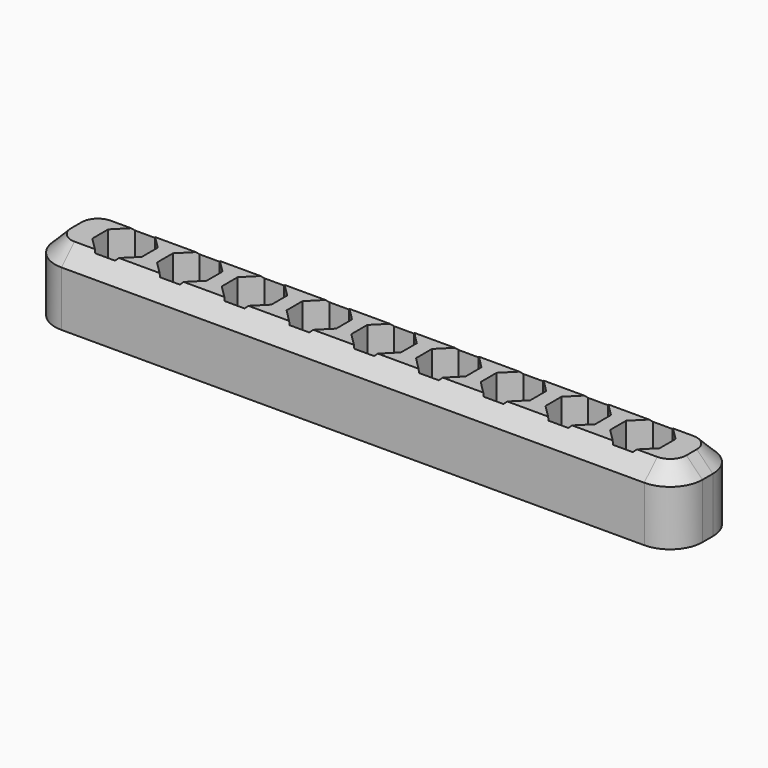
from build123d import *

# Parameters (mm, degrees)
F0_W         = 100
F0_H         = 12
F1_DEPTH     = 11
F0_W_2       = 2.3021356216
F0_H_2       = 3.0731172886
F0_W_3       = 3.0519974387
F0_H_3       = 2.2957974076
F2_DEPTH     = 1
F3_R         = 5
F4_T1_DEPTH  = 90
F4_T3_DEPTH  = 2
F4_T6_ANGLE  = 90
F4_T8_ANGLE  = 90
F4_T10_ANGLE = 90
F4_T12_ANGLE = 90


# Not quite as in the source:
# - a fillet or chamfer that OpenCascade refuses, or shapes differently, is made with other operations: its cross-section is extruded or revolved along the edge and cut away or added


with BuildPart() as f1:
    # F0 (on Top) → F1 (new body)
    with BuildSketch(Plane.XY):
        Rectangle(F0_W, F0_H)
        Polygon((-43.828134341, 1.5365586443), (-41.5259987194, 3.8323560519), (-38.4740012806, 3.8323560519), (-36.171865659, 1.5365586443), (-36.171865659, -1.5365586443), (-38.4740012806, -3.8323560519), (-41.5259987194, -3.8323560519), (-43.828134341, -1.5365586443), align=None, mode=Mode.SUBTRACT)
        Polygon((-13.8175263533, 1.5313583214), (-11.5153907317, 3.827155729), (-8.463393293, 3.827155729), (-6.1612576714, 1.5313583214), (-6.1612576714, -1.5417589672), (-8.463393293, -3.8375563748), (-11.5153907317, -3.8375563748), (-13.8175263533, -1.5417589672), align=None, mode=Mode.SUBTRACT)
        Polygon((6.1764764136, 1.531357914), (8.4786120352, 3.8271553215), (11.5306094739, 3.8271553215), (13.8327450955, 1.531357914), (13.8327450955, -1.5417593747), (11.5306094739, -3.8375567823), (8.4786120352, -3.8375567823), (6.1764764136, -1.5417593747), align=None, mode=Mode.SUBTRACT)
        Polygon((36.1682959368, 1.5178143587), (38.4704315585, 3.8136117663), (41.5224289972, 3.8136117663), (43.8245646188, 1.5178143587), (43.8245646188, -1.5553029299), (41.5224289972, -3.8511003375), (38.4704315585, -3.8511003375), (36.1682959368, -1.5553029299), align=None, mode=Mode.SUBTRACT)
        Polygon((-33.8281344609, 1.5365587602), (-31.5259988393, 3.8323561678), (-28.4740014006, 3.8323561678), (-26.1718657789, 1.5365587602), (-26.1718657789, -1.5365585284), (-28.4740014006, -3.832355936), (-31.5259988393, -3.832355936), (-33.8281344609, -1.5365585284), align=None, mode=Mode.SUBTRACT)
        Polygon((-23.8324813077, 1.5400278102), (-21.5303456861, 3.8358252178), (-18.4783482474, 3.8358252178), (-16.1762126258, 1.5400278102), (-16.1762126258, -1.5330894784), (-18.4783482474, -3.828886886), (-21.5303456861, -3.828886886), (-23.8324813077, -1.5330894784), align=None, mode=Mode.SUBTRACT)
        Polygon((-3.8348879394, 1.5600861226), (-1.5327523178, 3.8558835302), (1.5192451209, 3.8558835302), (3.8213807426, 1.5600861226), (3.8213807426, -1.513031166), (1.5192451209, -3.8088285736), (-1.5327523178, -3.8088285736), (-3.8348879394, -1.513031166), align=None, mode=Mode.SUBTRACT)
        Polygon((16.1591154059, 1.5457221845), (18.4612510276, 3.8415195921), (21.5132484663, 3.8415195921), (23.8153840879, 1.5457221845), (23.8153840879, -1.5273951041), (21.5132484663, -3.8231925117), (18.4612510276, -3.8231925117), (16.1591154059, -1.5273951041), align=None, mode=Mode.SUBTRACT)
        Polygon((26.1708870998, 1.5457229285), (28.4730227214, 3.8415203361), (31.5250201601, 3.8415203361), (33.8271557817, 1.5457229285), (33.8271557817, -1.5273943601), (31.5250201601, -3.8231917677), (28.4730227214, -3.8231917677), (26.1708870998, -1.5273943601), align=None, mode=Mode.SUBTRACT)
    extrude(amount=F1_DEPTH)

    # F0 (on Top) → F2 (join)
    with BuildSketch(Plane.XY):
        Rectangle(F0_W, F0_H)
        Polygon((-43.828134341, 1.5365586443), (-41.5259987194, 3.8323560519), (-38.4740012806, 3.8323560519), (-36.171865659, 1.5365586443), (-36.171865659, -1.5365586443), (-38.4740012806, -3.8323560519), (-41.5259987194, -3.8323560519), (-43.828134341, -1.5365586443), align=None, mode=Mode.SUBTRACT)
        Polygon((-13.8175263533, 1.5313583214), (-11.5153907317, 3.827155729), (-8.463393293, 3.827155729), (-6.1612576714, 1.5313583214), (-6.1612576714, -1.5417589672), (-8.463393293, -3.8375563748), (-11.5153907317, -3.8375563748), (-13.8175263533, -1.5417589672), align=None, mode=Mode.SUBTRACT)
        Polygon((6.1764764136, 1.531357914), (8.4786120352, 3.8271553215), (11.5306094739, 3.8271553215), (13.8327450955, 1.531357914), (13.8327450955, -1.5417593747), (11.5306094739, -3.8375567823), (8.4786120352, -3.8375567823), (6.1764764136, -1.5417593747), align=None, mode=Mode.SUBTRACT)
        Polygon((36.1682959368, 1.5178143587), (38.4704315585, 3.8136117663), (41.5224289972, 3.8136117663), (43.8245646188, 1.5178143587), (43.8245646188, -1.5553029299), (41.5224289972, -3.8511003375), (38.4704315585, -3.8511003375), (36.1682959368, -1.5553029299), align=None, mode=Mode.SUBTRACT)
        Polygon((-33.8281344609, 1.5365587602), (-31.5259988393, 3.8323561678), (-28.4740014006, 3.8323561678), (-26.1718657789, 1.5365587602), (-26.1718657789, -1.5365585284), (-28.4740014006, -3.832355936), (-31.5259988393, -3.832355936), (-33.8281344609, -1.5365585284), align=None, mode=Mode.SUBTRACT)
        Polygon((-23.8324813077, 1.5400278102), (-21.5303456861, 3.8358252178), (-18.4783482474, 3.8358252178), (-16.1762126258, 1.5400278102), (-16.1762126258, -1.5330894784), (-18.4783482474, -3.828886886), (-21.5303456861, -3.828886886), (-23.8324813077, -1.5330894784), align=None, mode=Mode.SUBTRACT)
        Polygon((-3.8348879394, 1.5600861226), (-1.5327523178, 3.8558835302), (1.5192451209, 3.8558835302), (3.8213807426, 1.5600861226), (3.8213807426, -1.513031166), (1.5192451209, -3.8088285736), (-1.5327523178, -3.8088285736), (-3.8348879394, -1.513031166), align=None, mode=Mode.SUBTRACT)
        Polygon((16.1591154059, 1.5457221845), (18.4612510276, 3.8415195921), (21.5132484663, 3.8415195921), (23.8153840879, 1.5457221845), (23.8153840879, -1.5273951041), (21.5132484663, -3.8231925117), (18.4612510276, -3.8231925117), (16.1591154059, -1.5273951041), align=None, mode=Mode.SUBTRACT)
        Polygon((26.1708870998, 1.5457229285), (28.4730227214, 3.8415203361), (31.5250201601, 3.8415203361), (33.8271557817, 1.5457229285), (33.8271557817, -1.5273943601), (31.5250201601, -3.8231917677), (28.4730227214, -3.8231917677), (26.1708870998, -1.5273943601), align=None, mode=Mode.SUBTRACT)
        with Locations((-42.6770665302, 0)):
            Rectangle(F0_W_2, F0_H_2)
        Polygon((-41.5259987194, 1.5365586443), (-41.5259987194, 3.8323560519), (-43.828134341, 1.5365586443), align=None)
        with Locations((-40, 2.6844573481)):
            Rectangle(F0_W_3, F0_H_3)
        Polygon((-41.5259987194, -3.8323560519), (-41.5259987194, -1.5365586443), (-43.828134341, -1.5365586443), align=None)
        with Locations((-40, -2.6844573481)):
            Rectangle(F0_W_3, F0_H_3)
        with Locations((-40, 0)):
            Rectangle(F0_W_3, F0_H_2)
        with Locations((-37.3229334698, 0)):
            Rectangle(F0_W_2, F0_H_2)
        Polygon((-36.171865659, 1.5365586443), (-38.4740012806, 3.8323560519), (-38.4740012806, 1.5365586443), align=None)
        Polygon((-36.171865659, -1.5365586443), (-38.4740012806, -1.5365586443), (-38.4740012806, -3.8323560519), align=None)
        Polygon((-31.5259988393, -3.832355936), (-31.5259988393, -1.5365585284), (-33.8281344609, -1.5365585284), align=None)
        with Locations((-32.6770666501, 1.159e-07)):
            Rectangle(F0_W_2, F0_H_2)
        Polygon((-31.5259988393, 1.5365587602), (-31.5259988393, 3.8323561678), (-33.8281344609, 1.5365587602), align=None)
        with Locations((-30.0000001199, 2.684457464)):
            Rectangle(F0_W_3, F0_H_3)
        Polygon((-26.1718657789, 1.5365587602), (-28.4740014006, 3.8323561678), (-28.4740014006, 1.5365587602), align=None)
        with Locations((-27.3229335898, 1.159e-07)):
            Rectangle(F0_W_2, F0_H_2)
        with Locations((-30.0000001199, 1.159e-07)):
            Rectangle(F0_W_3, F0_H_2)
        with Locations((-30.0000001199, -2.6844572322)):
            Rectangle(F0_W_3, F0_H_3)
        Polygon((-26.1718657789, -1.5365585284), (-28.4740014006, -1.5365585284), (-28.4740014006, -3.832355936), align=None)
        Polygon((-21.5303456861, -3.828886886), (-21.5303456861, -1.5330894784), (-23.8324813077, -1.5330894784), align=None)
        with Locations((-22.6814134969, 0.0034691659)):
            Rectangle(F0_W_2, F0_H_2)
        Polygon((-21.5303456861, 1.5400278102), (-21.5303456861, 3.8358252178), (-23.8324813077, 1.5400278102), align=None)
        with Locations((-20.0043469667, 2.687926514)):
            Rectangle(F0_W_3, F0_H_3)
        with Locations((-20.0043469667, 0.0034691659)):
            Rectangle(F0_W_3, F0_H_2)
        with Locations((-20.0043469667, -2.6809881822)):
            Rectangle(F0_W_3, F0_H_3)
        Polygon((-16.1762126258, -1.5330894784), (-18.4783482474, -1.5330894784), (-18.4783482474, -3.828886886), align=None)
        with Locations((-17.3272804366, 0.0034691659)):
            Rectangle(F0_W_2, F0_H_2)
        Polygon((-16.1762126258, 1.5400278102), (-18.4783482474, 3.8358252178), (-18.4783482474, 1.5400278102), align=None)
        Polygon((-11.5153907317, 1.5313583214), (-11.5153907317, 3.827155729), (-13.8175263533, 1.5313583214), align=None)
        with Locations((-12.6664585425, -0.0052003229)):
            Rectangle(F0_W_2, F0_H_2)
        Polygon((-11.5153907317, -3.8375563748), (-11.5153907317, -1.5417589672), (-13.8175263533, -1.5417589672), align=None)
        with Locations((-9.9893920124, -2.689657671)):
            Rectangle(F0_W_3, F0_H_3)
        with Locations((-9.9893920124, 2.6792570252)):
            Rectangle(F0_W_3, F0_H_3)
        with Locations((-7.3123254822, -0.0052003229)):
            Rectangle(F0_W_2, F0_H_2)
        Polygon((-6.1612576714, 1.5313583214), (-8.463393293, 3.827155729), (-8.463393293, 1.5313583214), align=None)
        Polygon((-6.1612576714, -1.5417589672), (-8.463393293, -1.5417589672), (-8.463393293, -3.8375563748), align=None)
        with Locations((-9.9893920124, -0.0052003229)):
            Rectangle(F0_W_3, F0_H_2)
        Polygon((-1.5327523178, 1.5600861226), (-1.5327523178, 3.8558835302), (-3.8348879394, 1.5600861226), align=None)
        with Locations((-0.0067535984, 2.7079848264)):
            Rectangle(F0_W_3, F0_H_3)
        Polygon((3.8213807426, 1.5600861226), (1.5192451209, 3.8558835302), (1.5192451209, 1.5600861226), align=None)
        with Locations((2.6703129317, 0.0235274783)):
            Rectangle(F0_W_2, F0_H_2)
        with Locations((-0.0067535984, 0.0235274783)):
            Rectangle(F0_W_3, F0_H_2)
        with Locations((-2.6838201286, 0.0235274783)):
            Rectangle(F0_W_2, F0_H_2)
        with Locations((-0.0067535984, -2.6609298698)):
            Rectangle(F0_W_3, F0_H_3)
        Polygon((3.8213807426, -1.513031166), (1.5192451209, -1.513031166), (1.5192451209, -3.8088285736), align=None)
        Polygon((-1.5327523178, -3.8088285736), (-1.5327523178, -1.513031166), (-3.8348879394, -1.513031166), align=None)
        with Locations((7.3275442244, -0.0052007304)):
            Rectangle(F0_W_2, F0_H_2)
        Polygon((8.4786120352, 1.531357914), (8.4786120352, 3.8271553215), (6.1764764136, 1.531357914), align=None)
        with Locations((10.0046107545, 2.6792566177)):
            Rectangle(F0_W_3, F0_H_3)
        Polygon((13.8327450955, 1.531357914), (11.5306094739, 3.8271553215), (11.5306094739, 1.531357914), align=None)
        with Locations((12.6816772847, -0.0052007304)):
            Rectangle(F0_W_2, F0_H_2)
        with Locations((10.0046107545, -0.0052007304)):
            Rectangle(F0_W_3, F0_H_2)
        Polygon((8.4786120352, -3.8375567823), (8.4786120352, -1.5417593747), (6.1764764136, -1.5417593747), align=None)
        with Locations((10.0046107545, -2.6896580785)):
            Rectangle(F0_W_3, F0_H_3)
        Polygon((13.8327450955, -1.5417593747), (11.5306094739, -1.5417593747), (11.5306094739, -3.8375567823), align=None)
        with Locations((17.3101832167, 0.0091635402)):
            Rectangle(F0_W_2, F0_H_2)
        Polygon((18.4612510276, -3.8231925117), (18.4612510276, -1.5273951041), (16.1591154059, -1.5273951041), align=None)
        with Locations((19.9872497469, -2.6752938079)):
            Rectangle(F0_W_3, F0_H_3)
        Polygon((23.8153840879, -1.5273951041), (21.5132484663, -1.5273951041), (21.5132484663, -3.8231925117), align=None)
        with Locations((22.6643162771, 0.0091635402)):
            Rectangle(F0_W_2, F0_H_2)
        with Locations((19.9872497469, 0.0091635402)):
            Rectangle(F0_W_3, F0_H_2)
        with Locations((19.9872497469, 2.6936208883)):
            Rectangle(F0_W_3, F0_H_3)
        Polygon((18.4612510276, 1.5457221845), (18.4612510276, 3.8415195921), (16.1591154059, 1.5457221845), align=None)
        Polygon((23.8153840879, 1.5457221845), (21.5132484663, 3.8415195921), (21.5132484663, 1.5457221845), align=None)
        Polygon((28.4730227214, 1.5457229285), (28.4730227214, 3.8415203361), (26.1708870998, 1.5457229285), align=None)
        with Locations((27.3219549106, 0.0091642842)):
            Rectangle(F0_W_2, F0_H_2)
        Polygon((28.4730227214, -3.8231917677), (28.4730227214, -1.5273943601), (26.1708870998, -1.5273943601), align=None)
        with Locations((29.9990214407, -2.6752930639)):
            Rectangle(F0_W_3, F0_H_3)
        with Locations((29.9990214407, 0.0091642842)):
            Rectangle(F0_W_3, F0_H_2)
        with Locations((29.9990214407, 2.6936216323)):
            Rectangle(F0_W_3, F0_H_3)
        Polygon((33.8271557817, 1.5457229285), (31.5250201601, 3.8415203361), (31.5250201601, 1.5457229285), align=None)
        with Locations((32.6760879709, 0.0091642842)):
            Rectangle(F0_W_2, F0_H_2)
        Polygon((33.8271557817, -1.5273943601), (31.5250201601, -1.5273943601), (31.5250201601, -3.8231917677), align=None)
        with Locations((37.3193637477, -0.0187442856)):
            Rectangle(F0_W_2, F0_H_2)
        Polygon((38.4704315585, -3.8511003375), (38.4704315585, -1.5553029299), (36.1682959368, -1.5553029299), align=None)
        with Locations((39.9964302778, -2.7032016337)):
            Rectangle(F0_W_3, F0_H_3)
        with Locations((42.673496808, -0.0187442856)):
            Rectangle(F0_W_2, F0_H_2)
        with Locations((39.9964302778, 2.6657130625)):
            Rectangle(F0_W_3, F0_H_3)
        Polygon((38.4704315585, 1.5178143587), (38.4704315585, 3.8136117663), (36.1682959368, 1.5178143587), align=None)
        with Locations((39.9964302778, -0.0187442856)):
            Rectangle(F0_W_3, F0_H_2)
        Polygon((43.8245646188, 1.5178143587), (41.5224289972, 3.8136117663), (41.5224289972, 1.5178143587), align=None)
        Polygon((43.8245646188, -1.5553029299), (41.5224289972, -1.5553029299), (41.5224289972, -3.8511003375), align=None)
    extrude(amount=F2_DEPTH)

    # F3
    f3_edges = [f1.edges().sort_by_distance(p)[0] for p in [
        (-50, 6, 5.5),
        (50, -6, 5.5),
        (50, 6, 5.5),
        (-50, -6, 5.5),
    ]]
    fillet(f3_edges, radius=F3_R)

    # F4: chamfer of 2.5 on 8 edges, made by hand

    # F4_s2 → F4_t1 (cut)
    with BuildSketch(Plane.YZ.offset(-45)):
        Polygon((-6, 8.5), (-3.5, 11), (-6, 11), align=None)
        Polygon((3.5, 11), (6, 8.5), (6, 11), align=None)
    extrude(amount=F4_T1_DEPTH, mode=Mode.SUBTRACT)

    # F4_s4 → F4_t3 (cut)
    with BuildSketch(Plane.XZ.offset(-1)):
        Polygon((-47.5, 11), (-50, 8.5), (-50, 11), align=None)
        Polygon((47.5, 11), (50, 8.5), (50, 11), align=None)
    extrude(amount=F4_T3_DEPTH, mode=Mode.SUBTRACT)

    # F4_s5 → F4_t6 (revolve, cut)
    with BuildSketch(Plane.YZ.offset(-45)):
        Polygon((-6, 8.5), (-3.5, 11), (-6, 11), align=None)
    revolve(axis=Axis((-45, -1, 11), (0, 0, -1)), revolution_arc=F4_T6_ANGLE, mode=Mode.SUBTRACT)

    # F4_s7 → F4_t8 (revolve, cut)
    with BuildSketch(Plane.YZ.offset(45)):
        Polygon((-6, 8.5), (-3.5, 11), (-6, 11), align=None)
    revolve(axis=Axis((45, -1, 11), (0, 0, 1)), revolution_arc=F4_T8_ANGLE, mode=Mode.SUBTRACT)

    # F4_s9 → F4_t10 (revolve, cut)
    with BuildSketch(Plane.YZ.offset(-45)):
        Polygon((3.5, 11), (6, 8.5), (6, 11), align=None)
    revolve(axis=Axis((-45, 1, 11), (0, 0, 1)), revolution_arc=F4_T10_ANGLE, mode=Mode.SUBTRACT)

    # F4_s11 → F4_t12 (revolve, cut)
    with BuildSketch(Plane.XZ.offset(-1)):
        Polygon((47.5, 11), (50, 8.5), (50, 11), align=None)
    revolve(axis=Axis((45, 1, 11), (0, 0, 1)), revolution_arc=F4_T12_ANGLE, mode=Mode.SUBTRACT)


solid = f1.part
